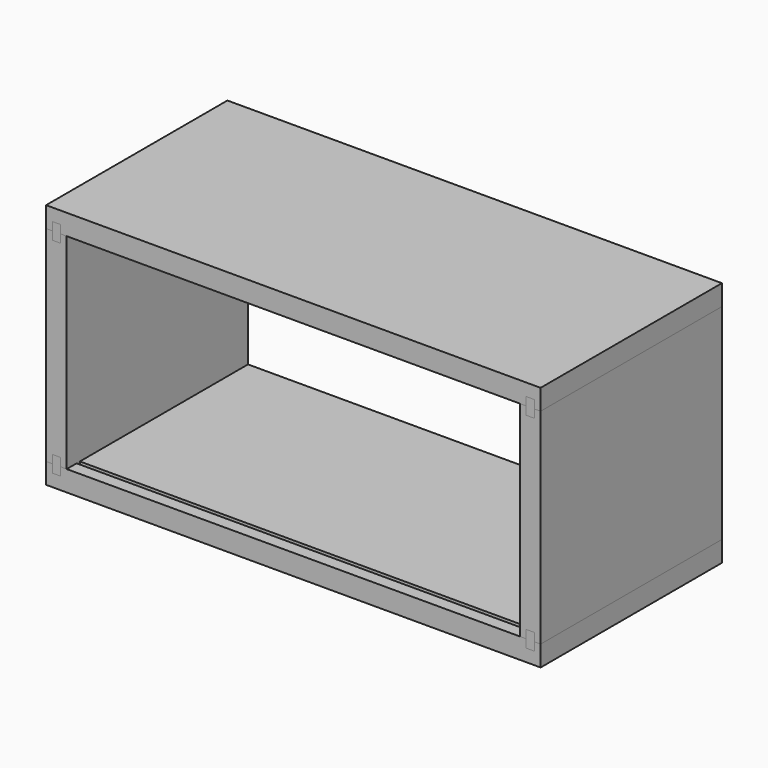
from build123d import *

# Parameters (mm, degrees)
F1_DEPTH  = 349.25
F2_DEPTH  = 349.25
F5_W      = 698.5
F5_H      = 6.35
F6_DEPTH  = 4.7625
F7_W      = 698.5
F7_H      = 6.35
F8_DEPTH  = 12.7
F10_DEPTH = 349.25


# Not quite as in the source:
# - a feature names something its author has since deleted; it is built from what else it names


with BuildPart() as f1:
    # F0 (on Front) → F1 (new body)
    with BuildSketch(Plane.XZ):
        Polygon((371.475, 157.95625), (381, 157.95625), (381, 189.70625), (-381, 189.70625), (-381, 157.95625), (-371.475, 157.95625), (-371.475, 170.65625), (-358.775, 170.65625), (-358.775, 157.95625), (-349.25, 157.95625), (349.25, 157.95625), (358.775, 157.95625), (358.775, 170.65625), (371.475, 170.65625), align=None)
    extrude(amount=-F1_DEPTH)


with BuildPart() as f2:
    # F0 (on Front) → F2 (new body)
    with BuildSketch(Plane.XZ):
        Polygon((-381, 157.95625), (-381, -157.95625), (-371.475, -157.95625), (-371.475, -145.25625), (-358.775, -145.25625), (-358.775, -157.95625), (-349.25, -157.95625), (-349.25, 157.95625), (-358.775, 157.95625), (-358.775, 145.25625), (-371.475, 145.25625), (-371.475, 157.95625), align=None)
    extrude(amount=-F2_DEPTH)


with BuildPart() as f3_1:
    # F3: instance of F1
    add(f1.part.mirror(Plane.XY))

    # F5 (on face) → F6 (cut)
    with BuildSketch(Plane.XY.offset(-157.95625)):
        with Locations((0, 22.225)):
            Rectangle(F5_W, F5_H)
    extrude(amount=-F6_DEPTH, mode=Mode.SUBTRACT)


with BuildPart() as f3_2:
    # F3: instance of F2
    add(f2.part.mirror(Plane.XY))


with BuildPart() as f4_1:
    # F4: instance of F2
    add(f2.part.mirror(Plane.YZ))


with BuildPart() as f1_1:
    add(f1.part)

    # F7 (on face) → F8 (cut)
    with BuildSketch(Plane(origin=(0, 0, 157.95625), x_dir=(1, 0, 0), z_dir=(0, 0, -1))):
        with Locations((0, -22.225)):
            Rectangle(F7_W, F7_H)
    extrude(amount=-F8_DEPTH, mode=Mode.SUBTRACT)


with BuildPart() as f10:
    # F9 (on face) → F10 (new body, through all)
    with BuildSketch(Plane.XZ):
        Polygon((-371.475, 170.65625), (-371.475, 157.95625), (-371.475, 145.25625), (-358.775, 145.25625), (-358.775, 157.95625), (-358.775, 170.65625), align=None)
    extrude(amount=-F10_DEPTH)


with BuildPart() as f11_1:
    # F11: instance of F10
    add(f10.part.mirror(Plane.YZ))


with BuildPart() as f12_1:
    # F12: instance of F10
    add(f10.part.mirror(Plane.XY))


with BuildPart() as f12_2:
    # F12: instance of F11_1
    add(f11_1.part.mirror(Plane.XY))


solid = Compound([f3_1.part, f3_2.part, f4_1.part, f1_1.part, f10.part, f11_1.part, f12_1.part, f12_2.part])
